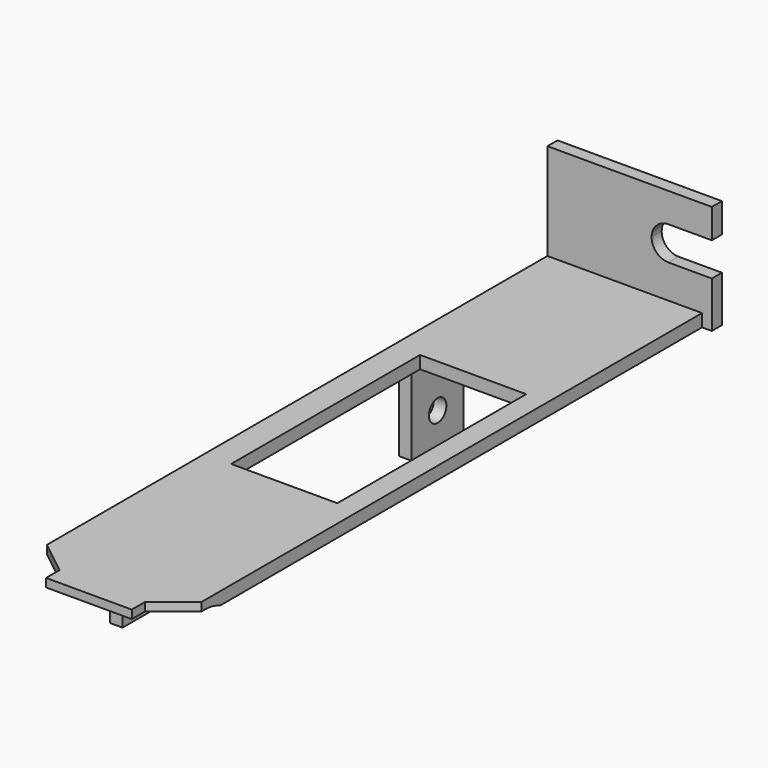
from build123d import *

# Parameters (mm, degrees)
F0_W         = 10.2
F0_H         = 2
F1_DEPTH     = 1.5
F2_W         = 12.64
F2_H         = 28.1
F3_DEPTH     = 25
F4_W         = 1.5
F4_H         = 75.9369339572
F5_DEPTH     = 10.5
F6_W         = 35.25
F6_H         = 10.5
F6_R         = 1.3
F6_W_2       = 15.825
F6_W_3       = 9.3619339572
F7_DEPTH     = 25
F9_DEPTH     = 0.5
F10_T1_DEPTH = 18.4
F11_W        = 18.4
F11_H        = 1.5
F11_W_2      = 1.1665335146
F12_DEPTH    = 11.5
F14_DEPTH    = 1.5
F15_DEPTH    = 1.5


# Not quite as in the source:
# - a fillet or chamfer that OpenCascade refuses, or shapes differently, is made with other operations: its cross-section is extruded or revolved along the edge and cut away or added


with BuildPart() as f1:
    # F0 (on Top) → F1 (new body)
    with BuildSketch(Plane.XY):
        Polygon((12.9583973216, 49.6379526287), (-5.4416026784, 49.6379526287), (-5.4416026784, -26.2989813285), (-1.3416026784, -29.5620473713), (8.8583973216, -29.5620473713), (12.9583973216, -26.2989813285), align=None)
        with Locations((3.7583973216, -30.5620473713)):
            Rectangle(F0_W, F0_H)
    extrude(amount=F1_DEPTH)

    # F2 (on face) → F3 (cut)
    with BuildSketch(Plane.XY.offset(1.5)):
        with Locations((4.0783973216, 11.1379526287)):
            Rectangle(F2_W, F2_H)
    extrude(amount=-F3_DEPTH, mode=Mode.SUBTRACT)

    # F4 (on face) → F5 (join)
    with BuildSketch(Plane(origin=(0, 0, 0), x_dir=(1, 0, 0), z_dir=(0, 0, -1))):
        with Locations((-4.6916026784, -11.6694856501)):
            Rectangle(F4_W, F4_H)
    extrude(amount=F5_DEPTH)

    # F6 (on face) → F7 (cut)
    with BuildSketch(Plane.YZ.offset(-3.9416026784)):
        with Locations((8.4379526287, -5.25)):
            Rectangle(F6_W, F6_H)
        with Locations((-13.0620473713, -6.8)):
            Circle(F6_R)
        with Locations((29.9379526287, -6.8)):
            Circle(F6_R)
        with Locations((41.7254526287, -5.25)):
            Rectangle(F6_W_2, F6_H)
        with Locations((-21.6180143499, -5.25)):
            Rectangle(F6_W_3, F6_H)
    extrude(amount=-F7_DEPTH, mode=Mode.SUBTRACT)

    # F8 (on face) → F9 (cut)
    with BuildSketch(Plane(origin=(0, 0, 0), x_dir=(1, 0, 0), z_dir=(0, 0, -1))):
        Polygon((-5.4416026784, 26.2989813285), (-5.4416026784, 23.5620473713), (12.9583973216, 23.5620473713), (12.9583973216, 26.2989813285), (8.8583973216, 29.5620473713), (8.8583973216, 31.5620473713), (-1.3416026784, 31.5620473713), (-1.3416026784, 29.5620473713), align=None)
    extrude(amount=-F9_DEPTH, mode=Mode.SUBTRACT)

    # F10: fillet of radius 5 on 1 edges, made by hand

    # F10_s2 → F10_t1 (join)
    with BuildSketch(Plane.YZ.offset(-5.4416026784)):
        with BuildLine():
            ThreePointArc((-25.7414968431, 0.5), (-24.6234628544, 0.3733971724), (-23.5620473713, 0))
            Line((-23.5620473713, 0), (-23.5620473713, 0.5))
            Line((-23.5620473713, 0.5), (-25.7414968431, 0.5))
        make_face()
    extrude(amount=F10_T1_DEPTH)

    # F11 (on face) → F12 (join)
    with BuildSketch(Plane.XY.offset(1.5)):
        with Locations((3.7583973216, 48.8879526287)):
            Rectangle(F11_W, F11_H)
        with Locations((13.5416640789, 48.8879526287)):
            Rectangle(F11_W_2, F11_H)
    extrude(amount=F12_DEPTH)

    # F13 (on face) → F14 (cut, through all)
    with BuildSketch(Plane(origin=(0, 49.6379526287, 0), x_dir=(-1, 0, 0), z_dir=(0, 1, 0))):
        with BuildLine():
            Line((-12.9583973216, 9.5), (-14.1249308363, 9.5))
            Line((-14.1249308363, 9.5), (-14.1249308363, 5.5))
            Line((-14.1249308363, 5.5), (-12.9583973216, 5.5))
            Line((-12.9583973216, 5.5), (-8.9583973216, 5.5))
            ThreePointArc((-8.9583973216, 5.5), (-10.9583973216, 7.5), (-8.9583973216, 9.5))
            Line((-8.9583973216, 9.5), (-12.9583973216, 9.5))
        make_face()
        with BuildLine():
            ThreePointArc((-6.9583973216, 7.5), (-7.5441837593, 8.9142135624), (-8.9583973216, 9.5))
            ThreePointArc((-8.9583973216, 9.5), (-10.9583973216, 7.5), (-8.9583973216, 5.5))
            ThreePointArc((-8.9583973216, 5.5), (-7.5441837593, 6.0857864376), (-6.9583973216, 7.5))
        make_face()
    extrude(amount=-F14_DEPTH, mode=Mode.SUBTRACT)

    # F15 (add, through all): a face of the model
    f15_faces = [f1.faces().sort_by_distance(p)[0] for p in [
        (13.5416640789, 48.8879526287, 1.5),
    ]]
    extrude(f15_faces, amount=F15_DEPTH)


solid = f1.part
